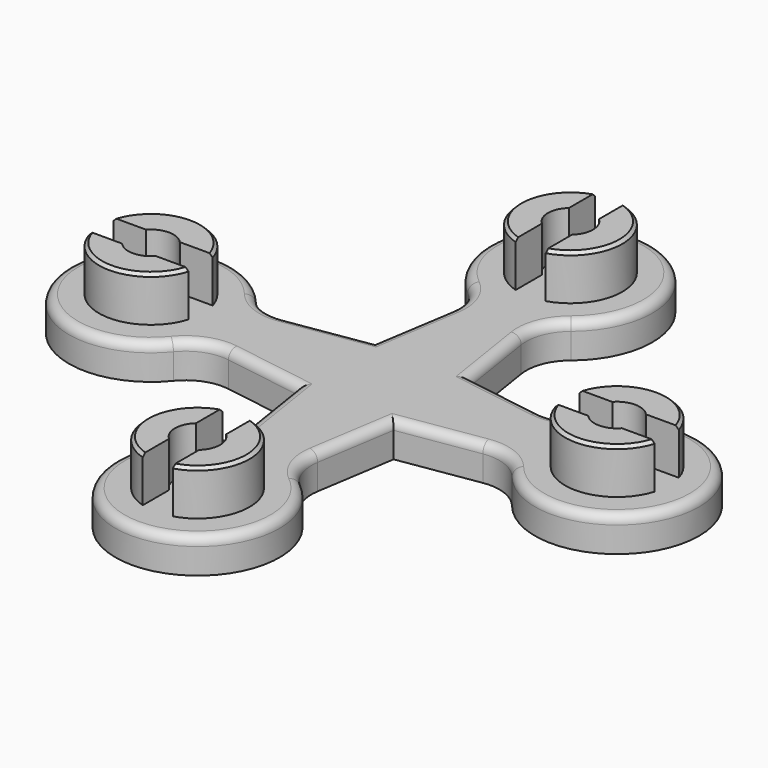
from build123d import *

# Parameters (mm, degrees)
F0_R     = 3.45
F1_DEPTH = 3
F2_SIZE  = 0.2
F4_DEPTH = 3
F6_COUNT = 4
F8_DEPTH = 2.3
F9_R     = 0.6


# Not quite as in the source:
# - a feature names something its author has since deleted; it is built from what else it names


with BuildPart() as f1:
    # F0 (on Top) → F1 (new body)
    with BuildSketch(Plane.XY):
        with Locations((0, 15.485)):
            Circle(F0_R)
    extrude(amount=F1_DEPTH)

    # F2
    f2_edges = [f1.edges().sort_by_distance(p)[0] for p in [
        (-3.45, 15.485, 3),
    ]]
    chamfer(f2_edges, length=F2_SIZE)

    # F3 (on face) → F4 (cut, through all)
    with BuildSketch(Plane.XY.offset(3)):
        with BuildLine():
            Line((-1, 19.435), (-1, 16.6030339887))
            ThreePointArc((-1, 16.6030339887), (-1.5, 15.485), (-1, 14.3669660113))
            Line((-1, 14.3669660113), (-1, 11.535))
            Line((-1, 11.535), (1, 11.535))
            Line((1, 11.535), (1, 14.3669660113))
            ThreePointArc((1, 14.3669660113), (1.5, 15.485), (1, 16.6030339887))
            Line((1, 16.6030339887), (1, 19.435))
            Line((1, 19.435), (-1, 19.435))
        make_face()
    extrude(amount=-F4_DEPTH, mode=Mode.SUBTRACT)


with BuildPart() as f6_1:
    # F6: instance of F1
    add(f1.part.rotate(Axis((0, 0, 1.3403603807), (0, 0, 1)), 1 * 360 / F6_COUNT))


with BuildPart() as f6_2:
    # F6: instance of F1
    add(f1.part.rotate(Axis((0, 0, 1.3403603807), (0, 0, 1)), 2 * 360 / F6_COUNT))


with BuildPart() as f6_3:
    # F6: instance of F1
    add(f1.part.rotate(Axis((0, 0, 1.3403603807), (0, 0, 1)), 3 * 360 / F6_COUNT))


with BuildPart() as f1_1:
    add(f1.part)

    add(f6_1.part)  # F8 merges F6_1

    add(f6_2.part)  # F8 merges F6_2

    add(f6_3.part)  # F8 merges F6_3
    # F7 (on Top) → F8 (join)
    with BuildSketch(Plane.XY):
        with BuildLine():
            ThreePointArc((2.3542748808, 8.4528817839), (2.5179079965, 9.995185414), (3.4299243827, 11.2496583693))
            ThreePointArc((3.4299243827, 11.2496583693), (0, 20.935), (-3.4299243827, 11.2496583693))
            ThreePointArc((-3.4299243827, 11.2496583693), (-2.5179079965, 9.995185414), (-2.3542748808, 8.4528817839))
            Line((-2.3542748808, 8.4528817839), (-3.1819805153, 3.1819805153))
            Line((-3.1819805153, 3.1819805153), (0, 4.5))
            Line((0, 4.5), (3.1819805153, 3.1819805153))
            Line((3.1819805153, 3.1819805153), (2.3542748808, 8.4528817839))
        make_face()
        Polygon((4.5, 0), (3.1819805153, 3.1819805153), (0, 4.5), (-3.1819805153, 3.1819805153), (-4.5, 0), (-3.1819805153, -3.1819805153), (0, -4.5), (3.1819805153, -3.1819805153), align=None)
        with BuildLine():
            Line((8.4528817839, 2.3542748808), (3.1819805153, 3.1819805153))
            Line((3.1819805153, 3.1819805153), (4.5, 0))
            Line((4.5, 0), (3.1819805153, -3.1819805153))
            Line((3.1819805153, -3.1819805153), (8.4528817839, -2.3542748808))
            ThreePointArc((8.4528817839, -2.3542748808), (9.995185414, -2.5179079965), (11.2496583693, -3.4299243827))
            ThreePointArc((11.2496583693, -3.4299243827), (20.935, 0), (11.2496583693, 3.4299243827))
            ThreePointArc((11.2496583693, 3.4299243827), (9.995185414, 2.5179079965), (8.4528817839, 2.3542748808))
        make_face()
        with BuildLine():
            Line((-4.5, 0), (-3.1819805153, 3.1819805153))
            Line((-3.1819805153, 3.1819805153), (-8.4528817839, 2.3542748808))
            ThreePointArc((-8.4528817839, 2.3542748808), (-9.995185414, 2.5179079965), (-11.2496583693, 3.4299243827))
            ThreePointArc((-11.2496583693, 3.4299243827), (-20.935, 0), (-11.2496583693, -3.4299243827))
            ThreePointArc((-11.2496583693, -3.4299243827), (-9.995185414, -2.5179079965), (-8.4528817839, -2.3542748808))
            Line((-8.4528817839, -2.3542748808), (-3.1819805153, -3.1819805153))
            Line((-3.1819805153, -3.1819805153), (-4.5, 0))
        make_face()
        with BuildLine():
            Line((2.3542748808, -8.4528817839), (3.1819805153, -3.1819805153))
            Line((3.1819805153, -3.1819805153), (0, -4.5))
            Line((0, -4.5), (-3.1819805153, -3.1819805153))
            Line((-3.1819805153, -3.1819805153), (-2.3542748808, -8.4528817839))
            ThreePointArc((-2.3542748808, -8.4528817839), (-2.5179079965, -9.995185414), (-3.4299243827, -11.2496583693))
            ThreePointArc((-3.4299243827, -11.2496583693), (0, -20.935), (3.4299243827, -11.2496583693))
            ThreePointArc((3.4299243827, -11.2496583693), (2.5179079965, -9.995185414), (2.3542748808, -8.4528817839))
        make_face()
    extrude(amount=-F8_DEPTH)

    # F9
    f9_edges = [f1_1.edges().sort_by_distance(p)[0] for p in [
        (2.768128, 5.817431, 0),
        (5.817431, 2.768128, 0),
        (2.517908, 9.995185, 0),
        (9.995185, 2.517908, 0),
        (0, 20.935, 0),
        (20.935, 0, 0),
        (-2.517908, 9.995185, 0),
        (9.995185, -2.517908, 0),
        (-2.768128, 5.817431, 0),
        (5.817431, -2.768128, 0),
        (-5.817431, 2.768128, 0),
        (2.768128, -5.817431, 0),
        (-9.995185, 2.517908, 0),
        (2.517908, -9.995185, 0),
        (-20.935, 0, 0),
        (0, -20.935, 0),
        (-9.995185, -2.517908, 0),
        (-2.517908, -9.995185, 0),
        (-5.817431, -2.768128, 0),
        (-2.768128, -5.817431, 0),
    ]]
    fillet(f9_edges, radius=F9_R)


solid = f1_1.part
